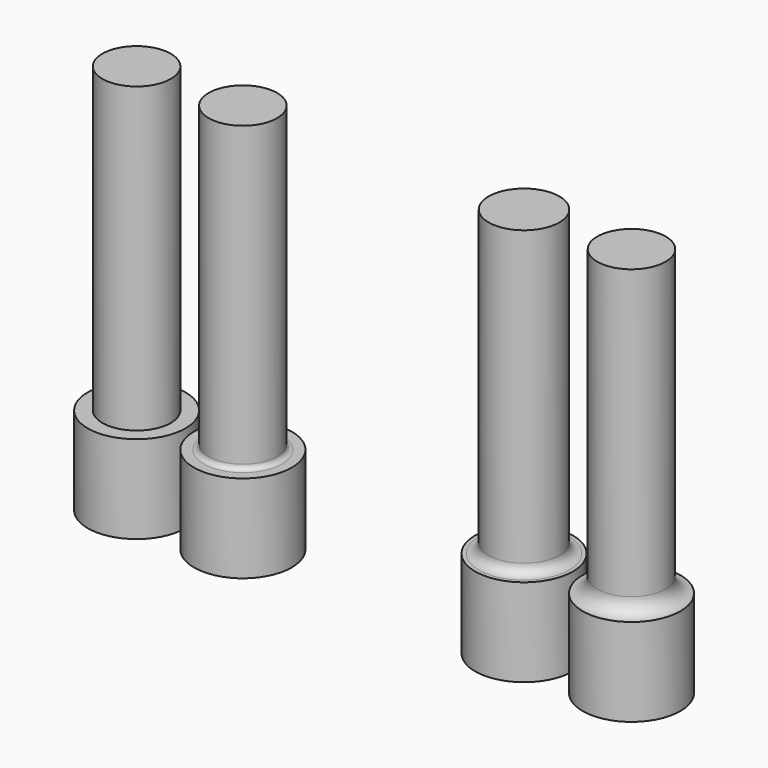
from build123d import *

# Parameters (mm, degrees)
F0_R     = 3.5
F1_DEPTH = 40
F0_R_2   = 3.6191233998
F2_R     = 5
F3_DEPTH = 9
F4_R     = 0.5
F5_R     = 1
F6_R     = 1.49999


# Not quite as in the source:
# - a fillet or chamfer is up to 0.001 mm smaller than in the source, because OpenCascade refuses the exact size


with BuildPart() as f1:
    # F0 (on Top) → F1 (new body)
    with BuildSketch(Plane.XY):
        with Locations((-9.4550363719, -10.4895196855)):
            Circle(F0_R)
    extrude(amount=F1_DEPTH)

    # F2 (on Top) → F3 (join)
    with BuildSketch(Plane.XY):
        with Locations((-9.4550363719, -10.4895196855)):
            Circle(F2_R)
    extrude(amount=F3_DEPTH)


with BuildPart() as f1b:
    # F0 (on Top) → F1, piece 2 (new body)
    with BuildSketch(Plane.XY):
        with Locations((1.4204620384, -10.4895196855)):
            Circle(F0_R)
    extrude(amount=F1_DEPTH)

    # F2 (on Top) → F3, piece 2 (join)
    with BuildSketch(Plane.XY):
        with Locations((1.4204620384, -10.4895196855)):
            Circle(F2_R)
    extrude(amount=F3_DEPTH)

    # F4
    f4_edges = [f1b.edges().sort_by_distance(p)[0] for p in [
        (-2.079538, -10.48952, 9),
    ]]
    fillet(f4_edges, radius=F4_R)


with BuildPart() as f1c:
    # F0 (on Top) → F1, piece 3 (new body)
    with BuildSketch(Plane.XY):
        with Locations((30.196333304, -10.4895196855)):
            Circle(F0_R_2)
    extrude(amount=F1_DEPTH)

    # F2 (on Top) → F3, piece 3 (join)
    with BuildSketch(Plane.XY):
        with Locations((30.196333304, -10.4895196855)):
            Circle(F2_R)
    extrude(amount=F3_DEPTH)

    # F5
    f5_edges = [f1c.edges().sort_by_distance(p)[0] for p in [
        (26.57721, -10.48952, 9),
    ]]
    fillet(f5_edges, radius=F5_R)


with BuildPart() as f1d:
    # F0 (on Top) → F1, piece 4 (new body)
    with BuildSketch(Plane.XY):
        with Locations((41.196333304, -10.4895196855)):
            Circle(F0_R)
    extrude(amount=F1_DEPTH)

    # F2 (on Top) → F3, piece 4 (join)
    with BuildSketch(Plane.XY):
        with Locations((41.196333304, -10.4895196855)):
            Circle(F2_R)
    extrude(amount=F3_DEPTH)

    # F6 (radius 1.5 in the source; OpenCascade refuses exactly that, so slightly less here)
    f6_edges = [f1d.edges().sort_by_distance(p)[0] for p in [
        (37.696333, -10.48952, 9),
    ]]
    fillet(f6_edges, radius=F6_R)


solid = Compound([f1.part, f1b.part, f1c.part, f1d.part])
